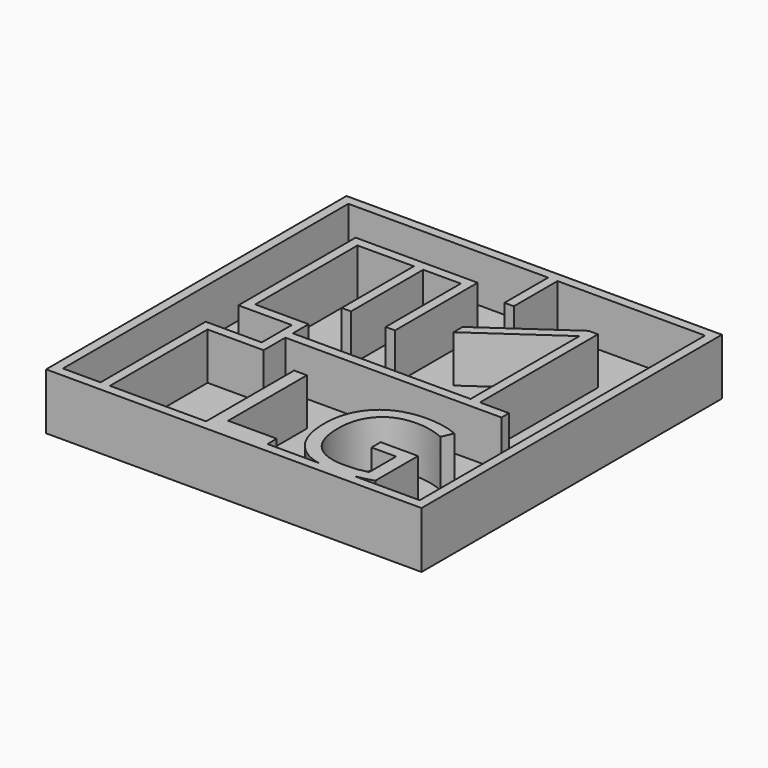
from build123d import *

# Parameters (mm, degrees)
F0_W          = 50.8
F0_H          = 50.8
F1_DEPTH      = 7.62
F2_T          = -1.27
F3_W          = 1.27
F3_H          = 17.78
F4_DEPTH      = 6.35
F5_W          = 7.5862407315
F5_H          = 1.27
F6_DEPTH      = 6.35
F7_W          = 1.27
F7_H          = 5.08
F8_DEPTH      = 6.35
F10_DEPTH     = 6.35
F12_R         = 1.27
F11_R         = 1.27
F13_DEPTH     = 25.4
F14_W         = 1.27
F14_H         = 17.290962553
F15_DEPTH     = 6.35
F17_DEPTH     = 6.35
F19_DEPTH     = 6.35
F20_TEXT_SIZE = 20.8606786761
F21_DEPTH     = 6.35
F22_R         = 1.27
F23_DEPTH     = 25.4
F24_R         = 1.27
F25_DEPTH     = 25.4
F27_DEPTH     = 6.35
F28_R         = 1.27
F29_DEPTH     = 25.4
F30_W         = 1.27
F30_H         = 12.7
F31_DEPTH     = 6.35
F32_W         = 1.27
F32_H         = 7.2665273991
F33_DEPTH     = 6.35
F34_R         = 1.27
F35_DEPTH     = 6.35
F36_DEPTH     = 25.4
F37_W         = 1.27
F37_H         = 12.210962553
F38_DEPTH     = 6.35
F39_W         = 1.27
F39_H         = 7.3849065221
F40_DEPTH     = 6.35
F41_DEPTH     = 10.5499543795
F42_W         = 5.08
F42_H         = 6.35
F43_DEPTH     = 25.4


# Not quite as in the source:
# - Text() gives the source's letters only with a copy of the font that has no kerning and outlines rounded to 1/6400 em; it was checked with that copy


with BuildPart() as f1:
    # F0 (on Top) → F1 (new body)
    with BuildSketch(Plane.XY):
        with Locations((-25.4, 25.4)):
            Rectangle(F0_W, F0_H)
    extrude(amount=F1_DEPTH)

    # F2
    f2_openings = [f1.faces().sort_by_distance(p)[0] for p in [
        (-25.4, 25.4, 7.62),
    ]]
    offset(amount=F2_T, openings=f2_openings)

    # F3 (on face) → F4 (join)
    with BuildSketch(Plane.XY.offset(1.27)):
        with Locations((-43.815, 10.16)):
            Rectangle(F3_W, F3_H)
    extrude(amount=F4_DEPTH)

    # F5 (on face) → F6 (join)
    with BuildSketch(Plane.XY.offset(1.27)):
        with Locations((-39.3868796343, 18.415)):
            Rectangle(F5_W, F5_H)
    extrude(amount=F6_DEPTH)

    # F7 (on face) → F8 (join)
    with BuildSketch(Plane.XY.offset(1.27)):
        with Locations((-36.2287592685, 21.59)):
            Rectangle(F7_W, F7_H)
    extrude(amount=F8_DEPTH)

    # F9 (on face) → F10 (join)
    with BuildSketch(Plane.XY.offset(1.27)):
        Polygon((-36.8637592685, 24.13), (-35.5937592685, 24.13), (-35.5937592685, 25.4), (-44.0879575908, 25.4), (-44.0879575908, 24.13), align=None)
    extrude(amount=F10_DEPTH)

    # F12 (on face) + F11 (on face) → F13 (cut)
    with BuildSketch(Plane.XY.offset(1.27)):
        with Locations((-46.99, 11.43)):
            Circle(F12_R)
    with BuildSketch(Plane.XY.offset(1.27)):
        with Locations((-46.99, 3.81)):
            Circle(F11_R)
    extrude(amount=-F13_DEPTH, mode=Mode.SUBTRACT)

    # F14 (on face) → F15 (join)
    with BuildSketch(Plane.XY.offset(1.27)):
        with Locations((-43.4529575908, 34.0454812765)):
            Rectangle(F14_W, F14_H)
    extrude(amount=F15_DEPTH)

    # F16 (on face) → F17 (join)
    with BuildSketch(Plane.XY.offset(1.27)):
        Polygon((-44.0879575908, 43.960962553), (-44.0879575908, 42.690962553), (-42.8179575908, 42.690962553), (-28.8479575908, 42.690962553), (-28.8479575908, 43.960962553), align=None)
    extrude(amount=F17_DEPTH)

    # F18 (on face) → F19 (join)
    with BuildSketch(Plane.XY.offset(1.27)):
        Polygon((-27.5779575908, 43.960962553), (-28.8479575908, 43.960962553), (-28.8479575908, 42.690962553), (-28.8479575908, 29.990962553), (-27.5779575908, 29.990962553), align=None)
    extrude(amount=F19_DEPTH)

    # F20 (on face) → F21 (join)
    with BuildSketch(Plane.XY.offset(1.27)):
        with Locations((-32.2162089595, 1.27)):
            Text('LG', F20_TEXT_SIZE, font='Open Sans', text_align=(TextAlign.LEFT, TextAlign.BOTTOM))
    extrude(amount=F21_DEPTH)

    # F22 (on face) → F23 (cut)
    with BuildSketch(Plane.XY.offset(1.27)):
        with Locations((-12.0017717973, 4.9849441218)):
            Circle(F22_R)
    extrude(amount=-F23_DEPTH, mode=Mode.SUBTRACT)

    # F24 (on face) → F25 (cut)
    with BuildSketch(Plane.XY.offset(1.27)):
        with Locations((-46.99, 19.05)):
            Circle(F24_R)
    extrude(amount=-F25_DEPTH, mode=Mode.SUBTRACT)

    # F26 (on face) → F27 (join)
    with BuildSketch(Plane.XY.offset(1.27)):
        Polygon((-27.5779575908, 31.5381352773), (-27.5779575908, 29.990962553), (-10.8235982352, 41.6484803694), (-11.5489470457, 42.690962553), align=None)
    extrude(amount=F27_DEPTH)

    # F28 (on face) → F29 (cut)
    with BuildSketch(Plane.XY.offset(1.27)):
        with Locations((-40.2779575908, 40.150962553)):
            Circle(F28_R)
    extrude(amount=-F29_DEPTH, mode=Mode.SUBTRACT)

    # F30 (on face) → F31 (join)
    with BuildSketch(Plane.XY.offset(1.27)):
        with Locations((-10.9139470457, 36.340962553)):
            Rectangle(F30_W, F30_H)
    extrude(amount=F31_DEPTH)

    # F32 (on face) → F33 (join)
    with BuildSketch(Plane.XY.offset(1.27)):
        Polygon((-6.35, 21.4544351539), (-6.35, 22.7244351539), (-10.2789470457, 22.7244351539), (-11.5489470457, 22.7244351539), (-25.043804889, 22.7244351539), (-25.043804889, 21.4544351539), align=None)
        with Locations((-10.9139470457, 26.3576988535)):
            Rectangle(F32_W, F32_H)
    extrude(amount=F33_DEPTH)

    # F34 (on face) → F35 (cut)
    with BuildSketch(Plane.XY.offset(1.27)):
        with Locations((-14.0889470457, 36.2821374588)):
            Circle(F34_R)
    extrude(amount=F35_DEPTH, mode=Mode.SUBTRACT)

    # F34 (on face) → F36 (cut)
    with BuildSketch(Plane.XY.offset(1.27)):
        with Locations((-14.0889470457, 36.2821374588)):
            Circle(F34_R)
    extrude(amount=-F36_DEPTH, mode=Mode.SUBTRACT)

    # F37 (on face) → F38 (join)
    with BuildSketch(Plane.XY.offset(1.27)):
        with Locations((-34.5629575908, 36.5854812765)):
            Rectangle(F37_W, F37_H)
    extrude(amount=F38_DEPTH)

    # F39 (on face) → F40 (join)
    with BuildSketch(Plane.XY.offset(1.27)):
        with Locations((-21.8629575908, 45.8375467389)):
            Rectangle(F39_W, F39_H)
    extrude(amount=F40_DEPTH)

    # F41 (add, through all): a face of the model
    f41_faces = [f1.faces().sort_by_distance(p)[0] for p in [
        (-25.043804889, 22.0894351539, 4.445),
    ]]
    extrude(f41_faces, amount=F41_DEPTH)

    # F42 (on face) → F43 (cut)
    with BuildSketch(Plane.XZ.offset(-49.53)):
        with Locations((-25.0379575908, 4.445)):
            Rectangle(F42_W, F42_H)
    extrude(amount=F43_DEPTH, mode=Mode.SUBTRACT)


solid = f1.part
